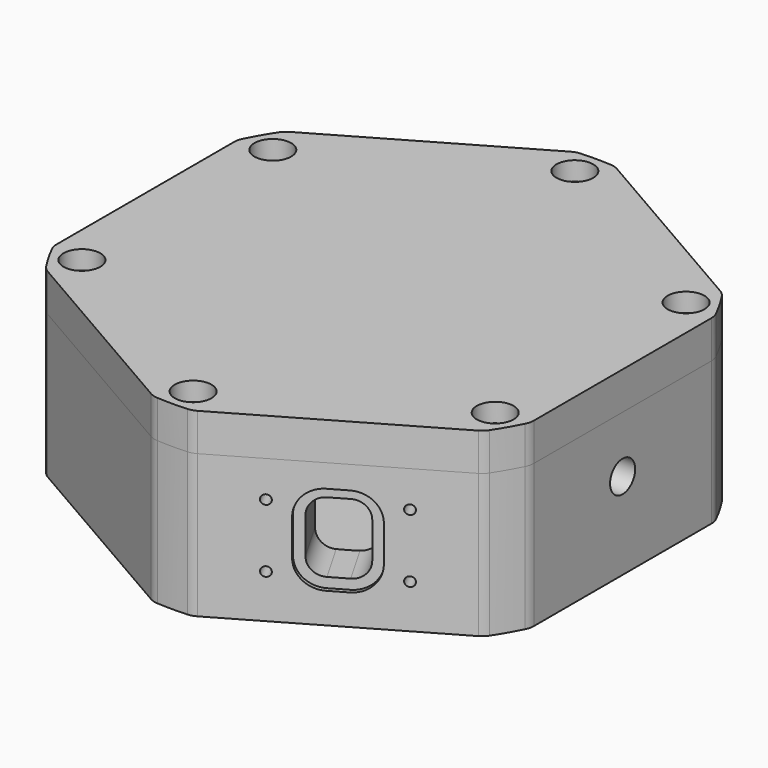
from build123d import *

# Parameters (mm, degrees)
F5_R            = 49.5
F6_DEPTH        = 30
F8_DEPTH        = 25
F11_DEPTH       = 8
F12_DEPTH       = 1.2
F13_D           = 2.5
F13_DEPTH       = 6.5
F13_TIP         = 0.7510757738
F14_D           = 8.33
F16_R           = 55.3
F16_R_2         = 52.2
F17_DEPTH       = 2
F19_D           = 4.2
F19_DEPTH       = 7.4
F19_TIP         = 1.2618073
F21_DEPTH       = 10
F23_D           = 5.5
F23_CBORE_D     = 9.75
F23_CBORE_DEPTH = 5
F24_R           = 5
F25_R           = 5
F26_D           = 2.5
F26_DEPTH       = 5
F26_TIP         = 0.7510757738


with BuildPart() as f6:
    # F5 (on Top) → F6 (new body)
    with BuildSketch(Plane.XY):
        with BuildLine():
            Line((-63.3, 30.5810398777), (-63.3, -30.5810398777))
            ThreePointArc((-63.3, -30.5810398777), (-60.881585886, -35.15), (-58.1339574082, -39.5288881207))
            Line((-58.1339574082, -39.5288881207), (-5.1660425918, -70.1099279984))
            ThreePointArc((-5.1660425918, -70.1099279984), (0, -70.3), (5.1660425918, -70.1099279984))
            Line((5.1660425918, -70.1099279984), (58.1339574082, -39.5288881207))
            ThreePointArc((58.1339574082, -39.5288881207), (60.881585886, -35.15), (63.3, -30.5810398777))
            Line((63.3, -30.5810398777), (63.3, 30.5810398777))
            ThreePointArc((63.3, 30.5810398777), (60.881585886, 35.15), (58.1339574082, 39.5288881207))
            Line((58.1339574082, 39.5288881207), (5.1660425918, 70.1099279984))
            ThreePointArc((5.1660425918, 70.1099279984), (0, 70.3), (-5.1660425918, 70.1099279984))
            Line((-5.1660425918, 70.1099279984), (-58.1339574082, 39.5288881207))
            ThreePointArc((-58.1339574082, 39.5288881207), (-60.881585886, 35.15), (-63.3, 30.5810398777))
        make_face()
        Circle(F5_R, mode=Mode.SUBTRACT)
    extrude(amount=F6_DEPTH)

    # F7 (on line) → F8 (cut)
    with BuildSketch(Plane(origin=(31.65, -54.8194080596, 0), x_dir=(0.8660254038, 0.5, 0), z_dir=(0.5, -0.8660254038, 0))):
        with BuildLine():
            Line((2.5, 21.3), (-2.5, 21.3))
            ThreePointArc((-2.5, 21.3), (-5.6819805153, 19.9819805153), (-7, 16.8))
            Line((-7, 16.8), (-7, 7.2))
            ThreePointArc((-7, 7.2), (-5.6819805153, 4.0180194847), (-2.5, 2.7))
            Line((-2.5, 2.7), (2.5, 2.7))
            ThreePointArc((2.5, 2.7), (5.6819805153, 4.0180194847), (7, 7.2))
            Line((7, 7.2), (7, 16.8))
            ThreePointArc((7, 16.8), (5.6819805153, 19.9819805153), (2.5, 21.3))
        make_face()
    extrude(amount=-F8_DEPTH, mode=Mode.SUBTRACT)

    # F10 (on Top) → F11 (join)
    with BuildSketch(Plane.XY):
        with BuildLine():
            Line((-63.3, 30.5810398777), (-63.3, -30.5810398777))
            ThreePointArc((-63.3, -30.5810398777), (-60.881585886, -35.15), (-58.1339574082, -39.5288881207))
            Line((-58.1339574082, -39.5288881207), (-5.1660425918, -70.1099279984))
            ThreePointArc((-5.1660425918, -70.1099279984), (0, -70.3), (5.1660425918, -70.1099279984))
            Line((5.1660425918, -70.1099279984), (58.1339574082, -39.5288881207))
            ThreePointArc((58.1339574082, -39.5288881207), (60.881585886, -35.15), (63.3, -30.5810398777))
            Line((63.3, -30.5810398777), (63.3, 30.5810398777))
            ThreePointArc((63.3, 30.5810398777), (60.881585886, 35.15), (58.1339574082, 39.5288881207))
            Line((58.1339574082, 39.5288881207), (5.1660425918, 70.1099279984))
            ThreePointArc((5.1660425918, 70.1099279984), (0, 70.3), (-5.1660425918, 70.1099279984))
            Line((-5.1660425918, 70.1099279984), (-58.1339574082, 39.5288881207))
            ThreePointArc((-58.1339574082, 39.5288881207), (-60.881585886, 35.15), (-63.3, 30.5810398777))
        make_face()
    extrude(amount=-F11_DEPTH)

    # F9 (on line) → F12 (cut)
    with BuildSketch(Plane(origin=(31.65, -54.8194080596, 0), x_dir=(0.8660254038, 0.5, 0), z_dir=(0.5, -0.8660254038, 0))):
        with BuildLine():
            Line((2.5, 23.92), (-2.5, 23.92))
            ThreePointArc((-2.5, 23.92), (-7.534600282, 21.834600282), (-9.62, 16.8))
            Line((-9.62, 16.8), (-9.62, 7.2))
            ThreePointArc((-9.62, 7.2), (-7.534600282, 2.165399718), (-2.5, 0.08))
            Line((-2.5, 0.08), (2.5, 0.08))
            ThreePointArc((2.5, 0.08), (7.534600282, 2.165399718), (9.62, 7.2))
            Line((9.62, 7.2), (9.62, 16.8))
            ThreePointArc((9.62, 16.8), (7.534600282, 21.834600282), (2.5, 23.92))
        make_face()
    extrude(amount=-F12_DEPTH, mode=Mode.SUBTRACT)

    # F13
    with Locations(Plane(origin=(31.65, -54.8194080596, 0), x_dir=(0.8660254038, 0.5, 0), z_dir=(0.5, -0.8660254038, 0))):
        with Locations((-15.1, 20.4), (-15.1, 3.6), (15.1, 3.6), (15.1, 20.4)):
            Hole(F13_D / 2, depth=F13_DEPTH)
            with Locations((0, 0, -(F13_DEPTH + F13_TIP / 2))):  # 118° drill point
                Cone(0, F13_D / 2, F13_TIP, mode=Mode.SUBTRACT)

    # F14 (through all)
    with Locations(Plane.YZ.offset(63.3)):
        with Locations((0, 15)):
            Hole(F14_D / 2)

    # F16 (on offset) → F17 (cut)
    with BuildSketch(Plane.XY.offset(30)):
        Circle(F16_R)
        Circle(F16_R_2, mode=Mode.SUBTRACT)
    extrude(amount=-F17_DEPTH, mode=Mode.SUBTRACT)

    # F19
    with Locations(Plane.XY.offset(30)):
        with Locations((-54.8194080596, -31.65), (0, -63.3), (54.8194080596, -31.65), (0, 63.3), (54.8194080596, 31.65), (-54.8194080596, 31.65)):
            Hole(F19_D / 2, depth=F19_DEPTH)
            with Locations((0, 0, -(F19_DEPTH + F19_TIP / 2))):  # 118° drill point
                Cone(0, F19_D / 2, F19_TIP, mode=Mode.SUBTRACT)

    # F25
    f25_edges = [f6.edges().sort_by_distance(p)[0] for p in [
        (5.166043, -70.109928, 11),
        (-5.166043, -70.109928, 11),
        (58.133957, -39.528888, 11),
        (63.3, -30.58104, 11),
        (63.3, 30.58104, 11),
        (58.133957, 39.528888, 11),
        (5.166043, 70.109928, 11),
        (-5.166043, 70.109928, 11),
        (-58.133957, 39.528888, 11),
        (-63.3, 30.58104, 11),
        (-63.3, -30.58104, 11),
        (-58.133957, -39.528888, 11),
    ]]
    fillet(f25_edges, radius=F25_R)

    # F26
    with Locations(Plane.XY):
        with Locations((-17.5, 39.5), (17.5, 39.5)):
            Hole(F26_D / 2, depth=F26_DEPTH)
            with Locations((0, 0, -(F26_DEPTH + F26_TIP / 2))):  # 118° drill point
                Cone(0, F26_D / 2, F26_TIP, mode=Mode.SUBTRACT)


with BuildPart() as f21:
    # F20 (on offset) → F21 (new body)
    with BuildSketch(Plane.XY.offset(30)):
        with BuildLine():
            Line((-5.1660425918, 70.1099279984), (-58.1339574082, 39.5288881207))
            ThreePointArc((-58.1339574082, 39.5288881207), (-60.881585886, 35.15), (-63.3, 30.5810398777))
            Line((-63.3, 30.5810398777), (-63.3, -30.5810398777))
            ThreePointArc((-63.3, -30.5810398777), (-60.881585886, -35.15), (-58.1339574082, -39.5288881207))
            Line((-58.1339574082, -39.5288881207), (-5.1660425918, -70.1099279984))
            ThreePointArc((-5.1660425918, -70.1099279984), (0, -70.3), (5.1660425918, -70.1099279984))
            Line((5.1660425918, -70.1099279984), (58.1339574082, -39.5288881207))
            ThreePointArc((58.1339574082, -39.5288881207), (60.881585886, -35.15), (63.3, -30.5810398777))
            Line((63.3, -30.5810398777), (63.3, 30.5810398777))
            ThreePointArc((63.3, 30.5810398777), (60.881585886, 35.15), (58.1339574082, 39.5288881207))
            Line((58.1339574082, 39.5288881207), (5.1660425918, 70.1099279984))
            ThreePointArc((5.1660425918, 70.1099279984), (0, 70.3), (-5.1660425918, 70.1099279984))
        make_face()
    extrude(amount=F21_DEPTH)

    # F23 (through all)
    with Locations(Plane.XY.offset(40)):
        with Locations((0, 63.3), (-54.8194080596, 31.65), (-54.8194080596, -31.65), (0, -63.3), (54.8194080596, -31.65), (54.8194080596, 31.65)):
            CounterBoreHole(F23_D / 2, F23_CBORE_D / 2, F23_CBORE_DEPTH)

    # F24
    f24_edges = [f21.edges().sort_by_distance(p)[0] for p in [
        (-58.133957, -39.528888, 35),
        (-63.3, -30.58104, 35),
        (5.166043, -70.109928, 35),
        (-5.166043, -70.109928, 35),
        (58.133957, -39.528888, 35),
        (63.3, -30.58104, 35),
        (63.3, 30.58104, 35),
        (58.133957, 39.528888, 35),
        (5.166043, 70.109928, 35),
        (-5.166043, 70.109928, 35),
        (-58.133957, 39.528888, 35),
        (-63.3, 30.58104, 35),
    ]]
    fillet(f24_edges, radius=F24_R)


solid = Compound([f6.part, f21.part])
